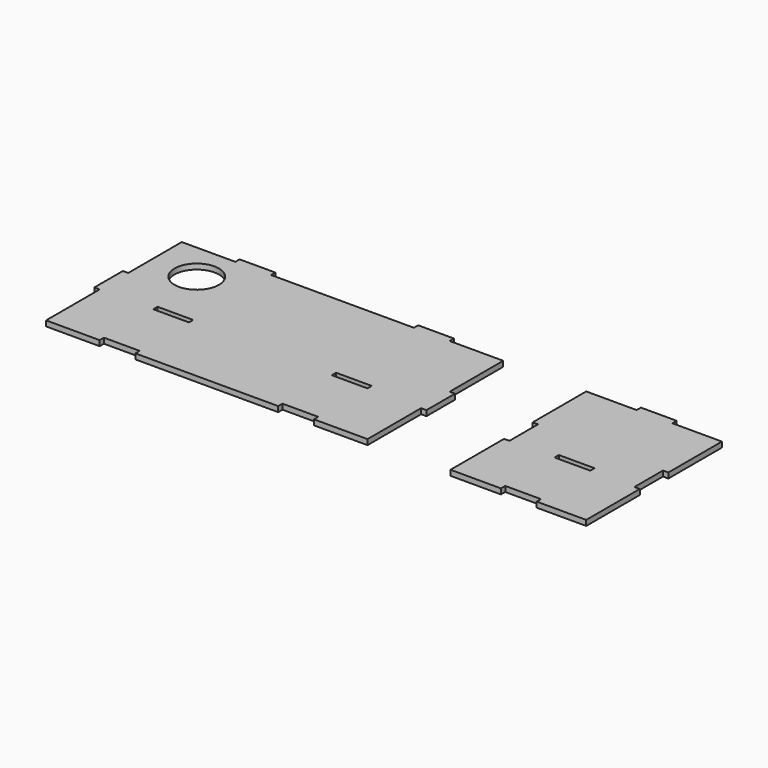
from build123d import *

# Parameters (mm, degrees)
F1_W     = 20
F1_H     = 3
F1_R     = 12.4378806179
F1_W_2   = 3
F1_H_2   = 20
F2_DEPTH = 3
F3_DEPTH = 3


# Not quite as in the source:
# - a feature names something its author has since deleted; it is built from what else it names


with BuildPart() as f2:
    # F1 (on Top) → F2 (new body)
    with BuildSketch(Plane.XY):
        Polygon((-90, -10), (-90, -47.5), (-60, -47.5), (-60, -44.5), (-40, -44.5), (-40, -47.5), (40, -47.5), (40, -44.5), (60, -44.5), (60, -47.5), (90, -47.5), (90, -10), (90, 10), (90, 47.5), (60, 47.5), (60, 50.5), (40, 50.5), (40, 47.5), (-40, 47.5), (-40, 50.5), (-60, 50.5), (-60, 47.5), (-90, 47.5), (-90, 10), align=None)
        with Locations((-50, -8.5)):
            Rectangle(F1_W, F1_H, mode=Mode.SUBTRACT)
        with Locations((50, -8.5)):
            Rectangle(F1_W, F1_H, mode=Mode.SUBTRACT)
        with Locations((-64.4147619605, 25.9968824685)):
            Circle(F1_R, mode=Mode.SUBTRACT)
        with Locations((91.5, 0)):
            Rectangle(F1_W_2, F1_H_2)
        with Locations((-91.5, 0)):
            Rectangle(F1_W_2, F1_H_2)
    extrude(amount=F2_DEPTH)


with BuildPart() as f3:
    # F1 (on Top) → F3 (new body)
    with BuildSketch(Plane.XY):
        Polygon((212.4768147469, -10), (209.4768147469, -10), (209.4768147469, 10), (212.4768147469, 10), (212.4768147469, 47.5), (184.7395757437, 47.5), (184.7395757437, 50.5), (164.7395757437, 50.5), (164.7395757437, 47.5), (136.4768147469, 47.5), (136.4768147469, 10), (139.4768147469, 10), (139.4768147469, -10), (136.4768147469, -10), (136.4768147469, -47.5), (164.7395757437, -47.5), (164.7395757437, -44.5), (184.7395757437, -44.5), (184.7395757437, -47.5), (212.4768147469, -47.5), align=None)
        with Locations((174.7395757437, -8.5)):
            Rectangle(F1_W, F1_H, mode=Mode.SUBTRACT)
    extrude(amount=F3_DEPTH)


solid = Compound([f2.part, f3.part])
